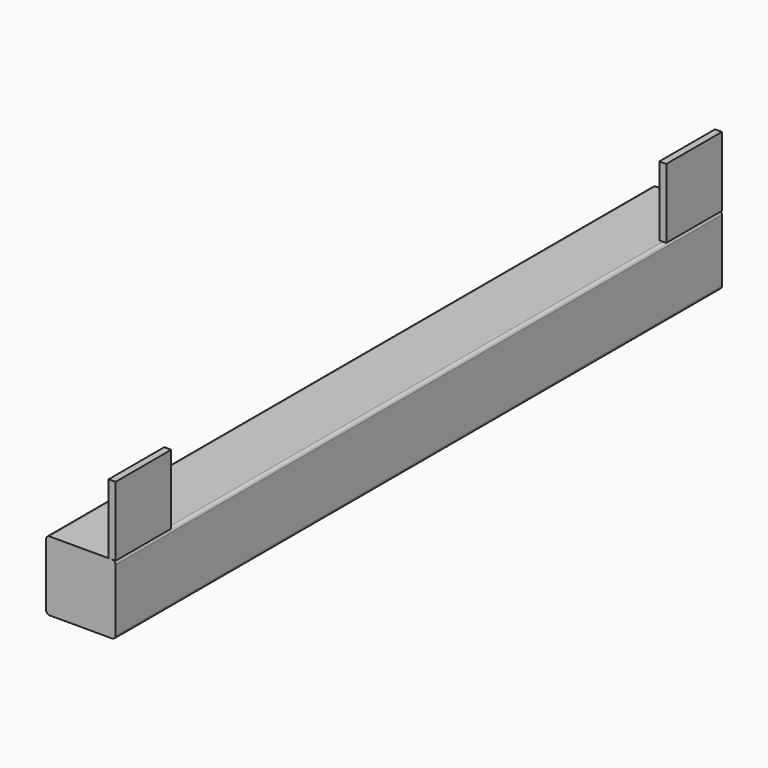
from build123d import *

# Parameters (mm, degrees)
F1_DEPTH  = 1078
F4_DEPTH  = 8
F7_DEPTH  = 6
F9_R      = 7
F10_DEPTH = 3
F11_W     = 90
F11_H     = 90
F11_R     = 6
F11_R_2   = 3
F12_DEPTH = 13
F13_W     = 5
F13_H     = 100
F14_DEPTH = 100


with BuildPart() as f1:
    # F0 (on Front) → F1 (new body)
    with BuildSketch(Plane.XZ):
        with BuildLine():
            ThreePointArc((50, 45), (48.5355339059, 48.5355339059), (45, 50))
            Line((45, 50), (-45, 50))
            ThreePointArc((-45, 50), (-48.5355339059, 48.5355339059), (-50, 45))
            Line((-50, 45), (-50, -45))
            ThreePointArc((-50, -45), (-48.5355339059, -48.5355339059), (-45, -50))
            Line((-45, -50), (45, -50))
            ThreePointArc((45, -50), (48.5355339059, -48.5355339059), (50, -45))
            Line((50, -45), (50, 45))
        make_face()
        with BuildLine():
            ThreePointArc((-47, 45), (-46.4142135624, 46.4142135624), (-45, 47))
            Line((-45, 47), (45, 47))
            ThreePointArc((45, 47), (46.4142135624, 46.4142135624), (47, 45))
            Line((47, 45), (47, -45))
            ThreePointArc((47, -45), (46.4142135624, -46.4142135624), (45, -47))
            Line((45, -47), (-45, -47))
            ThreePointArc((-45, -47), (-46.4142135624, -46.4142135624), (-47, -45))
            Line((-47, -45), (-47, 45))
        make_face(mode=Mode.SUBTRACT)
    extrude(amount=-F1_DEPTH)

    # F3 (on offset) → F4 (join)
    with BuildSketch(Plane.XZ.offset(6)):
        with BuildLine():
            ThreePointArc((50, 45), (48.5355339059, 48.5355339059), (45, 50))
            Line((45, 50), (-45, 50))
            ThreePointArc((-45, 50), (-48.5355339059, 48.5355339059), (-50, 45))
            Line((-50, 45), (-50, -45))
            ThreePointArc((-50, -45), (-48.5355339059, -48.5355339059), (-45, -50))
            Line((-45, -50), (45, -50))
            ThreePointArc((45, -50), (48.5355339059, -48.5355339059), (50, -45))
            Line((50, -45), (50, 45))
        make_face()
    extrude(amount=-F4_DEPTH)

    # F6 (on offset) → F7 (join)
    with BuildSketch(Plane(origin=(0, 1084, 0), x_dir=(-1, 0, 0), z_dir=(0, 1, 0))):
        with BuildLine():
            ThreePointArc((50, 45), (48.5355339059, 48.5355339059), (45, 50))
            Line((45, 50), (-45, 50))
            ThreePointArc((-45, 50), (-48.5355339059, 48.5355339059), (-50, 45))
            Line((-50, 45), (-50, -45))
            ThreePointArc((-50, -45), (-48.5355339059, -48.5355339059), (-45, -50))
            Line((-45, -50), (45, -50))
            ThreePointArc((45, -50), (48.5355339059, -48.5355339059), (50, -45))
            Line((50, -45), (50, 45))
        make_face()
    extrude(amount=-F7_DEPTH)

    # F8: union 

    # F9 (on face) → F10 (cut, through all)
    with BuildSketch(Plane(origin=(-50, 0, 0), x_dir=(0, -1, 0), z_dir=(-1, 0, 0))):
        with Locations((-784, 0)):
            Circle(F9_R)
        with Locations((-294, 0)):
            Circle(F9_R)
    extrude(amount=-F10_DEPTH, mode=Mode.SUBTRACT)

    # F11 (on face) → F12 (join)
    with BuildSketch(Plane.YZ.offset(50)):
        with Locations((1039, 0)):
            Rectangle(F11_W, F11_H)
        with Locations((1010, -29)):
            Circle(F11_R, mode=Mode.SUBTRACT)
        with Locations((1068, -29)):
            Circle(F11_R, mode=Mode.SUBTRACT)
        with Locations((1039, 0)):
            Circle(F11_R_2, mode=Mode.SUBTRACT)
        with Locations((1010, 29)):
            Circle(F11_R, mode=Mode.SUBTRACT)
        with Locations((1068, 29)):
            Circle(F11_R, mode=Mode.SUBTRACT)
        with Locations((39, 0)):
            Rectangle(F11_W, F11_H)
        with Locations((10, -29)):
            Circle(F11_R, mode=Mode.SUBTRACT)
        with Locations((68, -29)):
            Circle(F11_R, mode=Mode.SUBTRACT)
        with Locations((39, 0)):
            Circle(F11_R_2, mode=Mode.SUBTRACT)
        with Locations((10, 29)):
            Circle(F11_R, mode=Mode.SUBTRACT)
        with Locations((68, 29)):
            Circle(F11_R, mode=Mode.SUBTRACT)
    extrude(amount=-F12_DEPTH)

    # F13 (on face) → F14 (join)
    with BuildSketch(Plane.XY.offset(50)):
        with Locations((47.5, 1034)):
            Rectangle(F13_W, F13_H)
        with Locations((42.5, 1034)):
            Rectangle(F13_W, F13_H)
    extrude(amount=F14_DEPTH)


with BuildPart() as f14:
    # F13 (on face) → F14, piece 2 (new body)
    with BuildSketch(Plane.XY.offset(50)):
        with Locations((47.5, 44)):
            Rectangle(F13_W, F13_H)
        with Locations((42.5, 44)):
            Rectangle(F13_W, F13_H)
    extrude(amount=F14_DEPTH)


solid = Compound([f1.part, f14.part])
